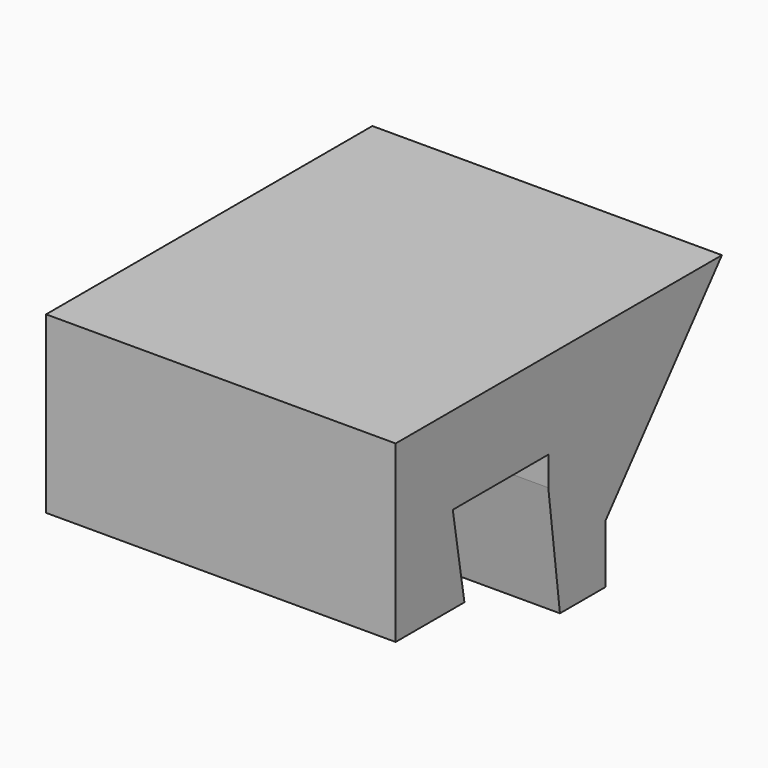
from build123d import *

# Parameters (mm, degrees)
F0_W     = 24
F0_H     = 4.9
F0_H_2   = 4.1
F1_DEPTH = 12
F2_DEPTH = 6
F3_DEPTH = 10
F4_SIZE2 = 11.99999
F4_SIZE  = 9.99999
F6_DEPTH = 24
F7_DEPTH = 4
F8_SIZE2 = 1
F8_SIZE  = 8


# Not quite as in the source:
# - a fillet or chamfer is up to 0.001 mm smaller than in the source, because OpenCascade refuses the exact size


with BuildPart() as f1:
    # F0 (on Top) → F1 (new body)
    with BuildSketch(Plane.XY):
        with Locations((-88, -2.45)):
            Rectangle(F0_W, F0_H)
        with Locations((-88, -6.95)):
            Rectangle(F0_W, F0_H_2)
        with Locations((-88, -11.05)):
            Rectangle(F0_W, F0_H_2)
        with Locations((-88, -15.55)):
            Rectangle(F0_W, F0_H)
    extrude(amount=F1_DEPTH)

    # F0 (on Top) → F2 (cut)
    with BuildSketch(Plane.XY):
        with Locations((-88, -6.95)):
            Rectangle(F0_W, F0_H_2)
        with Locations((-88, -11.05)):
            Rectangle(F0_W, F0_H_2)
    extrude(amount=F2_DEPTH, mode=Mode.SUBTRACT)

    # F3 (add): a face of the model
    f3_faces = [f1.faces().sort_by_distance(p)[0] for p in [
        (-88, 0, 6),
    ]]
    extrude(f3_faces, amount=F3_DEPTH)

    # F4 (size 10 and 12 in the source; OpenCascade refuses exactly that, so slightly less here)
    f4_edges = [f1.edges().sort_by_distance(p)[0] for p in [
        (-88, 10, 0),
    ]]
    f4_side = f1.faces().sort_by_distance((-88, 2.55, 0))[0]
    chamfer(f4_edges, length=F4_SIZE, length2=F4_SIZE2, reference=f4_side)

    # F5 (on face) → F6 (join, through all)
    with BuildSketch(Plane.YZ.offset(-76)):
        Polygon((-13.1, 0), (-12.1, 0), (-13.1, 6), align=None)
    extrude(amount=-F6_DEPTH)

    # F7 (add): a face of the model
    f7_faces = [f1.faces().sort_by_distance(p)[0] for p in [
        (-88, -2.449995, 0),
    ]]
    extrude(f7_faces, amount=F7_DEPTH)

    # F8
    f8_edges = [f1.edges().sort_by_distance(p)[0] for p in [
        (-88, -4.9, -4),
    ]]
    f8_side = f1.faces().sort_by_distance((-88, -4.9, 1))[0]
    chamfer(f8_edges, length=F8_SIZE, length2=F8_SIZE2, reference=f8_side)


solid = f1.part
